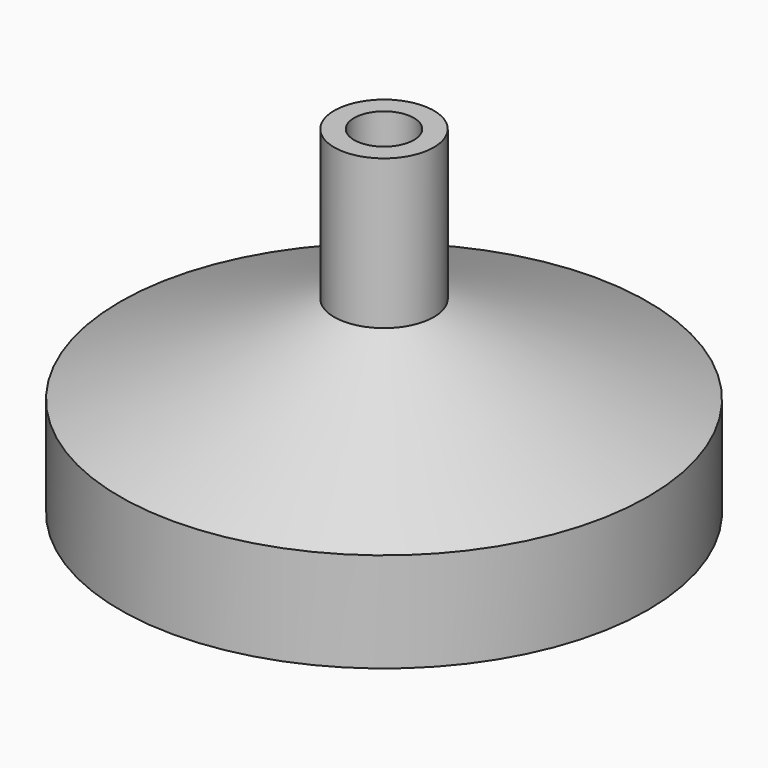
from build123d import *

# Parameters (mm, degrees)
F2_T = -2


# Not quite as in the source:
# - the program builds the solid bodies; features that only make, move or delete a surface that nothing else refers to are left out


with BuildPart() as f1:
    # F0 (on Right) → F1 (revolve)
    with BuildSketch(Plane.YZ):
        Polygon((0, 15.9718455747), (-5, 15.9718455747), (-5, 0.9718455747), (-26.5, -7.9165611044), (-26.5, -17.9165611044), (0, -17.9165611044), align=None)
    revolve(axis=Axis((0, 0, -0.4027476534), (0, 0, -1)))

    # F2
    f2_openings = [f1.faces().sort_by_distance(p)[0] for p in [
        (0, 0, -17.916561),
        (0, 0, 15.971846),
    ]]
    offset(amount=F2_T, openings=f2_openings, kind=Kind.INTERSECTION)


solid = f1.part
